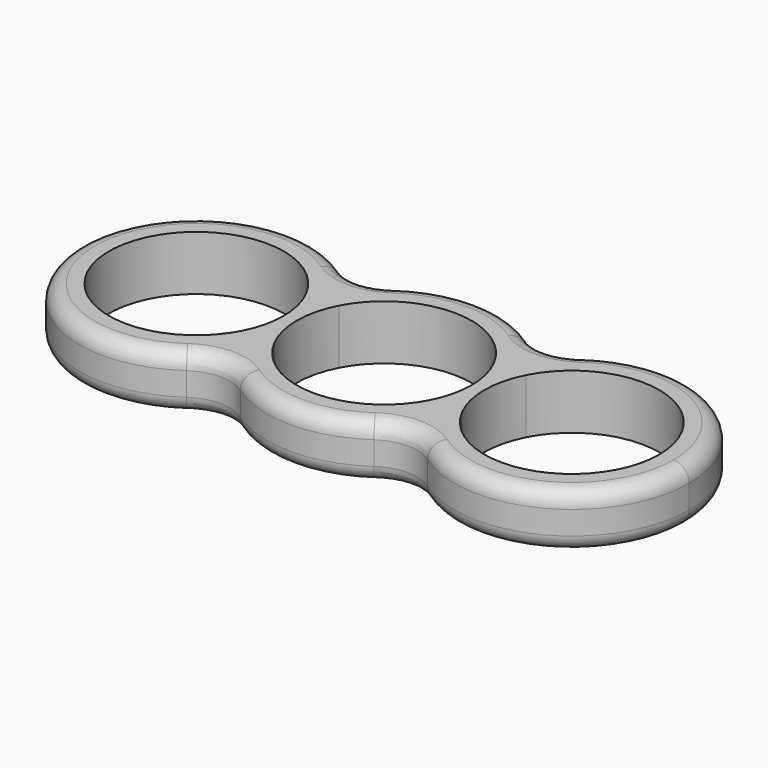
from build123d import *

# Parameters (mm, degrees)
F1_DEPTH = 7
F2_R     = 6
F3_R     = 2


# Not quite as in the source:
# - a feature names something its author has since deleted; it is built from what else it names


with BuildPart() as f1:
    # F0 (on Top) → F1 (new body)
    with BuildSketch(Plane.XY):
        with BuildLine():
            ThreePointArc((-14.0623969756, 5.1112299037), (-13.1615738007, 7.1167868393), (-11.9765766631, 8.9686839202))
            ThreePointArc((-11.9765766631, 8.9686839202), (-39, 0), (-11.9765766631, -8.9686839202))
            ThreePointArc((-11.9765766631, -8.9686839202), (-13.1615738007, -7.1167868393), (-14.0623969756, -5.1112299037))
            ThreePointArc((-14.0623969756, -5.1112299037), (-35.175, 0), (-14.0623969756, 5.1112299037))
        make_face()
        with BuildLine():
            ThreePointArc((-9.9141796875, -5.1565168597), (-11.175, 0), (-9.9141796875, 5.1565168597))
            ThreePointArc((-9.9141796875, 5.1565168597), (-10.8069599633, 7.1374851726), (-11.9765766631, 8.9686839202))
            ThreePointArc((-11.9765766631, 8.9686839202), (-13.1615738007, 7.1167868393), (-14.0623969756, 5.1112299037))
            ThreePointArc((-14.0623969756, 5.1112299037), (-13.1387537824, 2.6294401687), (-12.825, 0))
            ThreePointArc((-12.825, 0), (-13.1387537824, -2.6294401687), (-14.0623969756, -5.1112299037))
            ThreePointArc((-14.0623969756, -5.1112299037), (-13.1615738007, -7.1167868393), (-11.9765766631, -8.9686839202))
            ThreePointArc((-11.9765766631, -8.9686839202), (-10.8069599633, -7.1374851726), (-9.9141796875, -5.1565168597))
        make_face()
        with BuildLine():
            ThreePointArc((-9.9141796875, 5.1565168597), (0, 11.175), (9.9141796875, 5.1565168597))
            ThreePointArc((9.9141796875, 5.1565168597), (10.8069599633, 7.1374851726), (11.9765766631, 8.9686839202))
            ThreePointArc((11.9765766631, 8.9686839202), (0, 14.9624757252), (-11.9765766631, 8.9686839202))
            ThreePointArc((-11.9765766631, 8.9686839202), (-10.8069599633, 7.1374851726), (-9.9141796875, 5.1565168597))
        make_face()
        with BuildLine():
            ThreePointArc((9.9141796875, 5.1565168597), (10.8552195512, 2.6542105222), (11.175, 0))
            ThreePointArc((11.175, 0), (10.8552195512, -2.6542105222), (9.9141796875, -5.1565168597))
            ThreePointArc((9.9141796875, -5.1565168597), (10.8069599633, -7.1374851726), (11.9765766631, -8.9686839202))
            ThreePointArc((11.9765766631, -8.9686839202), (13.1615738007, -7.1167868393), (14.0623969756, -5.1112299037))
            ThreePointArc((14.0623969756, -5.1112299037), (12.825, 0), (14.0623969756, 5.1112299037))
            ThreePointArc((14.0623969756, 5.1112299037), (13.1615738007, 7.1167868393), (11.9765766631, 8.9686839202))
            ThreePointArc((11.9765766631, 8.9686839202), (10.8069599633, 7.1374851726), (9.9141796875, 5.1565168597))
        make_face()
        with BuildLine():
            ThreePointArc((39, 0), (28.724862429, 14.2364207239), (11.9765766631, 8.9686839202))
            ThreePointArc((11.9765766631, 8.9686839202), (13.1615738007, 7.1167868393), (14.0623969756, 5.1112299037))
            ThreePointArc((14.0623969756, 5.1112299037), (26.6294401687, 10.8612462176), (35.175, 0))
            ThreePointArc((35.175, 0), (26.6294401687, -10.8612462176), (14.0623969756, -5.1112299037))
            ThreePointArc((14.0623969756, -5.1112299037), (13.1615738007, -7.1167868393), (11.9765766631, -8.9686839202))
            ThreePointArc((11.9765766631, -8.9686839202), (28.724862429, -14.2364207239), (39, 0))
        make_face()
        with BuildLine():
            ThreePointArc((11.9765766631, -8.9686839202), (10.8069599633, -7.1374851726), (9.9141796875, -5.1565168597))
            ThreePointArc((9.9141796875, -5.1565168597), (0, -11.175), (-9.9141796875, -5.1565168597))
            ThreePointArc((-9.9141796875, -5.1565168597), (-10.8069599633, -7.1374851726), (-11.9765766631, -8.9686839202))
            ThreePointArc((-11.9765766631, -8.9686839202), (0, -14.9624757252), (11.9765766631, -8.9686839202))
        make_face()
    extrude(amount=F1_DEPTH)

    # F2
    f2_edges = [f1.edges().sort_by_distance(p)[0] for p in [
        (-11.976577, -8.968684, 3.5),
        (11.976577, -8.968684, 3.5),
        (11.976577, 8.968684, 3.5),
        (-11.976577, 8.968684, 3.5),
    ]]
    fillet(f2_edges, radius=F2_R)

    # F3
    f3_edges = [f1.edges().sort_by_distance(p)[0] for p in [
        (-39, 0, 7),
        (-39, 0, 0),
    ]]
    fillet(f3_edges, radius=F3_R)


solid = f1.part
